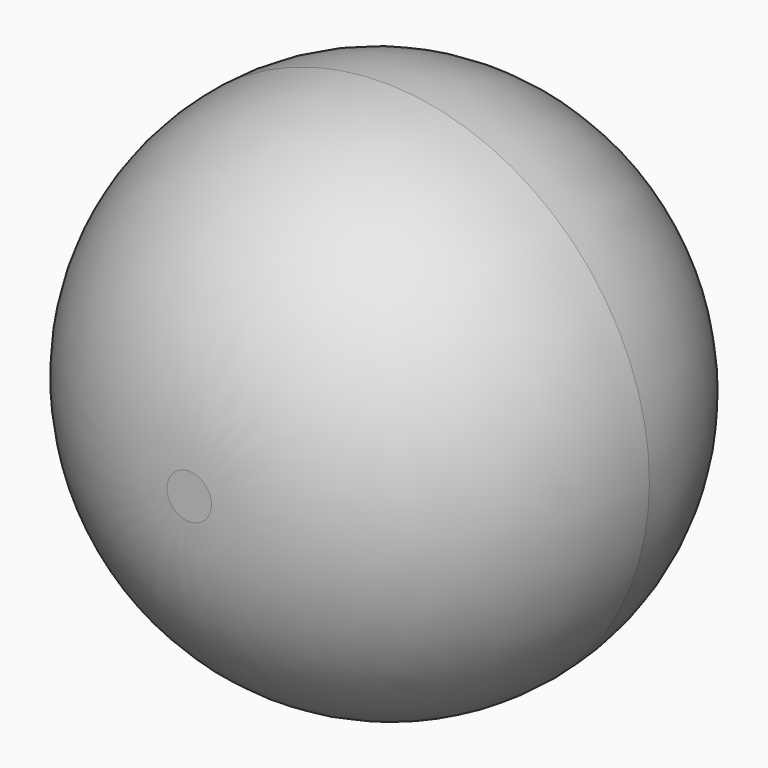
from build123d import *

# Parameters (mm, degrees)
F0_R     = 27.2834758809
F1_DEPTH = 25
F2_R     = 24.99999
F3_DEPTH = 25
F4_R     = 25


# Not quite as in the source:
# - a fillet or chamfer is up to 0.001 mm smaller than in the source, because OpenCascade refuses the exact size


with BuildPart() as f1:
    # F0 (on Front) → F1 (new body)
    with BuildSketch(Plane.XZ):
        Circle(F0_R)
    extrude(amount=F1_DEPTH)

    # F2 (radius 25 in the source; OpenCascade refuses exactly that, so slightly less here)
    f2_edges = [f1.edges().sort_by_distance(p)[0] for p in [
        (-27.283476, 0, 0),
    ]]
    fillet(f2_edges, radius=F2_R)

    # F3 (add): a face of the model
    f3_faces = [f1.faces().sort_by_distance(p)[0] for p in [
        (0, -25, 0),
    ]]
    extrude(f3_faces, amount=F3_DEPTH)

    # F4
    f4_edges = [f1.edges().sort_by_distance(p)[0] for p in [
        (-27.283476, -50, 0),
    ]]
    fillet(f4_edges, radius=F4_R)


solid = f1.part
